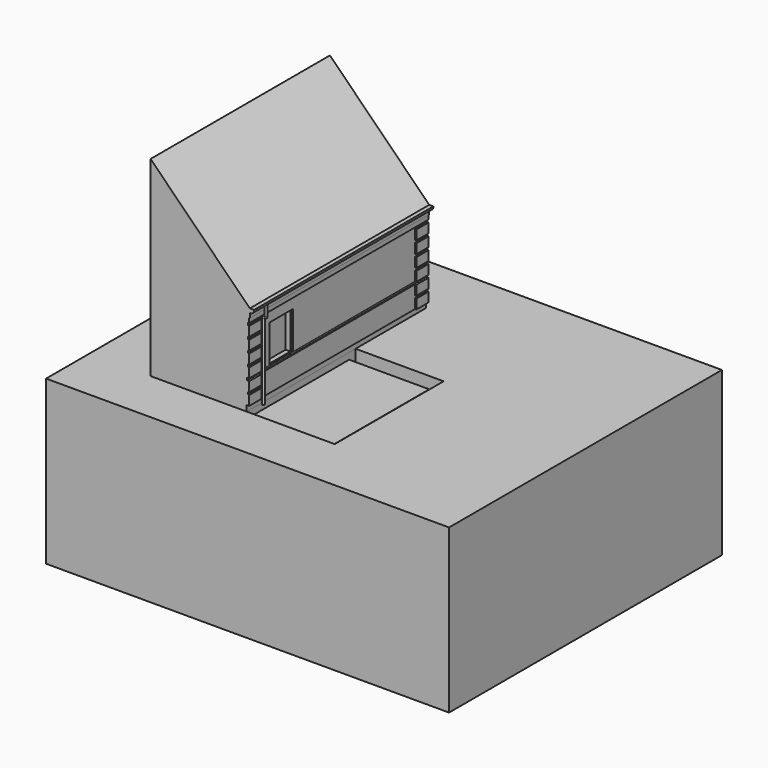
from build123d import *

# Parameters (mm, degrees)
F1_DEPTH  = 7000
F2_W      = 6040
F2_H      = 2460
F3_DEPTH  = 40
F6_R      = 37.5
F8_W      = 910
F8_H      = 1200
F9_DEPTH  = 200
F10_W     = 910
F10_H     = 1200
F10_W_2   = 830
F10_H_2   = 1140
F11_DEPTH = 150
F12_W     = 12582.5710296631
F12_H     = 10649.8882770538
F12_W_2   = 3000
F12_H_2   = 7000
F13_DEPTH = 5090
F14_W     = 2500
F14_H     = 4000
F15_DEPTH = 200
F14_H_2   = 250
F16_DEPTH = 900


# Not quite as in the source:
# - a feature names something its author has since deleted; it is built from what else it names


with BuildPart() as f1:
    # F0 (on Front) → F1 (new body)
    with BuildSketch(Plane.XZ):
        with BuildLine():
            Line((0, 180), (80, 180))
            Line((80, 180), (80, 480))
            Line((80, 480), (40, 480))
            Line((40, 480), (40, 560))
            Line((40, 560), (80, 560))
            Line((80, 560), (80, 860))
            Line((80, 860), (10, 860))
            Line((10, 860), (10, 940))
            Line((10, 940), (80, 940))
            Line((80, 940), (80, 1240))
            Line((80, 1240), (40, 1240))
            Line((40, 1240), (40, 1320))
            Line((40, 1320), (80, 1320))
            Line((80, 1320), (80, 1620))
            Line((80, 1620), (40, 1620))
            Line((40, 1620), (40, 1700))
            Line((40, 1700), (80, 1700))
            Line((80, 1700), (80, 2000))
            Line((80, 2000), (40, 2000))
            Line((40, 2000), (40, 2080))
            Line((40, 2080), (80, 2080))
            Line((80, 2080), (80, 2380))
            Line((80, 2380), (40, 2380))
            Line((40, 2380), (40, 2460))
            Line((40, 2460), (80, 2460))
            Line((80, 2460), (80, 2600))
            Line((80, 2600), (100, 2600))
            Line((100, 2600), (100, 2740))
            Line((100, 2740), (110, 2740))
            ThreePointArc((110, 2740), (194.8528137424, 2775.1471862576), (230, 2860))
            Line((230, 2860), (230, 2870))
            Line((230, 2870), (100, 2870))
            Line((100, 2870), (-3000, 5970))
            Line((-3000, 5970), (-3000, 0))
            Line((-3000, 0), (0, 0))
            Line((0, 0), (0, 180))
        make_face()
    extrude(amount=-F1_DEPTH)

    # F2 (on face) → F3 (cut, through all)
    with BuildSketch(Plane.YZ.offset(80)):
        with Locations((3500, 1230)):
            Rectangle(F2_W, F2_H)
    extrude(amount=-F3_DEPTH, mode=Mode.SUBTRACT)

    # F7: sweep along a path in F5
    with BuildLine(Plane(origin=(0, 555, 0), x_dir=(-1, 0, 0), z_dir=(0, 1, 0))) as f7_path:
        Line((-165, 2870), (-165, 2450))
        ThreePointArc((-165, 2450), (-153.2842712475, 2421.7157287525), (-125, 2410))
        Line((-125, 2410), (-120, 2410))
        ThreePointArc((-120, 2410), (-91.7157287525, 2398.2842712475), (-80, 2370))
        Line((-80, 2370), (-80, 0))
    # F6 (on face) → F7 (sweep)
    with BuildSketch(Plane(origin=(0, 0, 0), x_dir=(1, 0, 0), z_dir=(0, 0, -1))):
        with Locations((80, -555)):
            Circle(F6_R)
    sweep(path=f7_path.line)

    # F8 (on face) → F9 (cut)
    with BuildSketch(Plane.YZ.offset(40)):
        with Locations((1305, 1520)):
            Rectangle(F8_W, F8_H)
    extrude(amount=-F9_DEPTH, mode=Mode.SUBTRACT)

    # F10 (on face) → F11 (join)
    with BuildSketch(Plane.YZ.offset(-160)):
        with Locations((1305, 1520)):
            Rectangle(F10_W, F10_H)
        with Locations((1305, 1520)):
            Rectangle(F10_W_2, F10_H_2, mode=Mode.SUBTRACT)
    extrude(amount=F11_DEPTH)


with BuildPart() as f13:
    # F12 (on face) → F13 (new body)
    with BuildSketch(Plane(origin=(0, 0, 0), x_dir=(1, 0, 0), z_dir=(0, 0, -1))):
        with Locations((1383.4552764893, -3630.9741735458)):
            Rectangle(F12_W, F12_H)
        with Locations((-1500, -3500)):
            Rectangle(F12_W_2, F12_H_2, mode=Mode.SUBTRACT)
        with Locations((-1500, -3500)):
            Rectangle(F12_W_2, F12_H_2)
    extrude(amount=F13_DEPTH)

    # F14 (on face) → F15 (cut)
    with BuildSketch(Plane.XY):
        with Locations((1250, 2000)):
            Rectangle(F14_W, F14_H)
    extrude(amount=-F15_DEPTH, mode=Mode.SUBTRACT)

    # F14 (on face) → F16 (cut)
    with BuildSketch(Plane.XY):
        Polygon((2500, 4000), (2500, 0), (2750, 0), (2750, 4250), (2500, 4250), align=None)
        with Locations((1250, 4125)):
            Rectangle(F14_W, F14_H_2)
    extrude(amount=-F16_DEPTH, mode=Mode.SUBTRACT)


solid = Compound([f1.part, f13.part])
